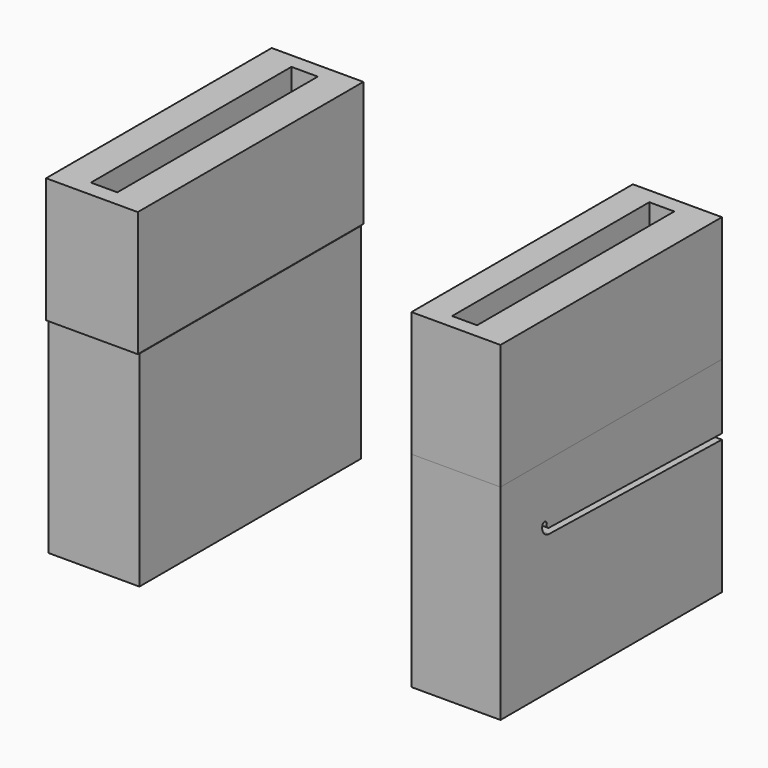
from build123d import *

# Parameters (mm, degrees)
F0_W     = 11.2702250481
F0_H     = 34.278973937
F0_W_2   = 8.2472413778
F0_H_2   = 30.5292597041
F1_DEPTH = 25.4
F0_W_3   = 11.0276525375
F0_W_4   = 7.7818950522
F2_DEPTH = 17.272
F3_W     = 11.0276525375
F3_H     = 34.278973937
F3_W_2   = 2.629864437
F3_H_2   = 30.5292597041
F3_W_3   = 2.0548701286
F4_DEPTH = 15.494
F3_W_4   = 11.3562569022
F3_H_3   = 34.9290966988
F3_W_5   = 3.269225359
F3_H_4   = 31.0449050739
F6_DEPTH = 59.182


with BuildPart() as f1:
    # F0 (on Top) → F1 (new body)
    with BuildSketch(Plane.XY):
        with Locations((-49.3858940899, 5.1079085097)):
            Rectangle(F0_W, F0_H)
        with Locations((-49.5420247316, 5.0395322032)):
            Rectangle(F0_W_2, F0_H_2, mode=Mode.SUBTRACT)
    extrude(amount=F1_DEPTH)


with BuildPart() as f1b:
    # F0 (on Top) → F1, piece 2 (new body)
    with BuildSketch(Plane.XY):
        with Locations((-4.5396565692, 5.1079085097)):
            Rectangle(F0_W_3, F0_H)
        with Locations((-4.6319066605, 5.0395322032)):
            Rectangle(F0_W_4, F0_H_2, mode=Mode.SUBTRACT)
    extrude(amount=F1_DEPTH)

    # F5 (on face) → F6 (cut)
    with BuildSketch(Plane.YZ.offset(0.9741696995)):
        with BuildLine():
            Line((-4.5115595148, 17.2269957008), (22.2473954782, 16.6359301656))
            Line((22.2473954782, 16.6359301656), (22.2473954782, 17.3218974883))
            Line((22.2473954782, 17.3218974883), (-4.4964149055, 17.9126285015))
            ThreePointArc((-4.4964149055, 17.9126285015), (-4.8215182289, 18.0877108855), (-4.870465867, 18.453702881))
            ThreePointArc((-4.870465867, 18.453702881), (-5.106187809, 18.8163662832), (-5.5172423918, 18.6817419644))
            ThreePointArc((-5.5172423918, 18.6817419644), (-5.3856405338, 17.6977266272), (-4.5115595148, 17.2269957008))
        make_face()
    extrude(amount=-F6_DEPTH, mode=Mode.SUBTRACT)


with BuildPart() as f2:
    # F0 (on Top) → F2 (new body)
    with BuildSketch(Plane.XY):
        with Locations((-4.6319066605, 5.0395322032)):
            Rectangle(F0_W_4, F0_H_2)
    extrude(amount=F2_DEPTH)


with BuildPart() as f2b:
    # F0 (on Top) → F2, piece 2 (new body)
    with BuildSketch(Plane.XY):
        with Locations((-49.5420247316, 5.0395322032)):
            Rectangle(F0_W_2, F0_H_2)
    extrude(amount=F2_DEPTH)


with BuildPart() as f4:
    # F3 (on face) → F4 (new body)
    with BuildSketch(Plane.XY.offset(25.4)):
        with Locations((-4.5396565692, 5.1079085097)):
            Rectangle(F3_W, F3_H)
        Polygon((-8.5228541866, 20.3041620553), (-6.467984058, 20.3041620553), (-3.3708235715, 20.3041620553), (-0.7409591344, 20.3041620553), (-0.7409591344, -10.2250976488), (-3.3708235715, -10.2250976488), (-6.467984058, -10.2250976488), (-8.5228541866, -10.2250976488), align=None, mode=Mode.SUBTRACT)
        with Locations((-2.0558913529, 5.0395322032)):
            Rectangle(F3_W_2, F3_H_2)
        with Locations((-7.4954191223, 5.0395322032)):
            Rectangle(F3_W_3, F3_H_2)
    extrude(amount=F4_DEPTH)


with BuildPart() as f4b:
    # F3 (on face) → F4, piece 2 (new body)
    with BuildSketch(Plane.XY.offset(25.4)):
        with Locations((-49.4841150939, 5.2479691803)):
            Rectangle(F3_W_4, F3_H_3)
        with Locations((-49.5701469481, 5.2973548882)):
            Rectangle(F3_W_5, F3_H_4, mode=Mode.SUBTRACT)
    extrude(amount=F4_DEPTH)


solid = Compound([f1.part, f1b.part, f2.part, f2b.part, f4.part, f4b.part])
